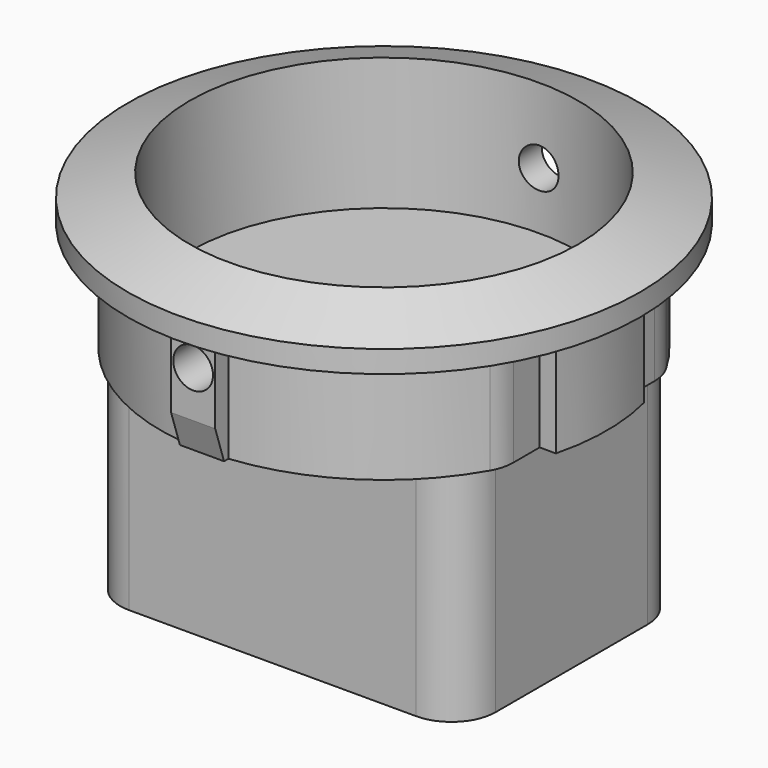
from build123d import *

# Parameters (mm, degrees)
F0_R      = 11.6
F1_DEPTH  = 2
F3_DEPTH  = 5
F5_DEPTH  = 10
F6_W      = 0.8
F6_H      = 5
F7_DEPTH  = 5
F8_R      = 8.8
F9_DEPTH  = 6
F10_SIZE2 = 0.99999
F10_SIZE  = 2.79999
F11_R     = 2
F12_SIZE2 = 0.5
F12_SIZE  = 1.5
F13_R     = 0.9
F14_DEPTH = 22.4013731274


# Not quite as in the source:
# - a fillet or chamfer is up to 0.001 mm smaller than in the source, because OpenCascade refuses the exact size


with BuildPart() as f1:
    # F0 (on Top) → F1 (new body)
    with BuildSketch(Plane.XY):
        Circle(F0_R)
    extrude(amount=F1_DEPTH)

    # F2 (on face) → F3 (join)
    with BuildSketch(Plane(origin=(0, 0, 0), x_dir=(1, 0, 0), z_dir=(0, 0, -1))):
        with BuildLine():
            Line((-9.05, -2.5), (-9.05, -4.4841387133))
            ThreePointArc((-9.05, -4.4841387133), (0, -10.1), (9.05, -4.4841387133))
            Line((9.05, -4.4841387133), (9.05, -2.5))
            Line((9.05, -2.5), (9.05, 2.5))
            Line((9.05, 2.5), (9.05, 4.4841387133))
            ThreePointArc((9.05, 4.4841387133), (5.7442463725, 8.3074444694), (1, 10.0503731274))
            Line((1, 10.0503731274), (1, 10.8003731274))
            Line((1, 10.8003731274), (-1, 10.8003731274))
            Line((-1, 10.8003731274), (-1, 10.0503731274))
            ThreePointArc((-1, 10.0503731274), (-5.7442463725, 8.3074444694), (-9.05, 4.4841387133))
            Line((-9.05, 4.4841387133), (-9.05, 2.5))
            Line((-9.05, 2.5), (-9.05, -2.5))
        make_face()
        with BuildLine():
            Line((-9.7857038582, -2.5), (-9.05, -2.5))
            Line((-9.05, -2.5), (-9.05, 2.5))
            Line((-9.05, 2.5), (-9.7857038582, 2.5))
            ThreePointArc((-9.7857038582, 2.5), (-10.1, 0), (-9.7857038582, -2.5))
        make_face()
        with BuildLine():
            Line((9.05, 2.5), (9.05, -2.5))
            Line((9.05, -2.5), (9.7857038582, -2.5))
            ThreePointArc((9.7857038582, -2.5), (10.1, 0), (9.7857038582, 2.5))
            Line((9.7857038582, 2.5), (9.05, 2.5))
        make_face()
    extrude(amount=F3_DEPTH)

    # F4 (on face) → F5 (join)
    with BuildSketch(Plane(origin=(0, 0, -5), x_dir=(1, 0, 0), z_dir=(0, 0, -1))):
        with BuildLine():
            Line((6.5, 6.3), (-6.5, 6.3))
            ThreePointArc((-6.5, 6.3), (-7.9142135624, 5.7142135624), (-8.5, 4.3))
            Line((-8.5, 4.3), (-8.5, -4.3))
            ThreePointArc((-8.5, -4.3), (-7.9142135624, -5.7142135624), (-6.5, -6.3))
            Line((-6.5, -6.3), (6.5, -6.3))
            ThreePointArc((6.5, -6.3), (7.9142135624, -5.7142135624), (8.5, -4.3))
            Line((8.5, -4.3), (8.5, 4.3))
            ThreePointArc((8.5, 4.3), (7.9142135624, 5.7142135624), (6.5, 6.3))
        make_face()
    extrude(amount=F5_DEPTH)

    # F6 (on face) → F7 (cut)
    with BuildSketch(Plane(origin=(0, 0, -15), x_dir=(1, 0, 0), z_dir=(0, 0, -1))):
        Rectangle(F6_W, F6_H)
        with Locations((-7.35, 0)):
            Rectangle(F6_W, F6_H)
        with Locations((7.35, 0)):
            Rectangle(F6_W, F6_H)
    extrude(amount=-F7_DEPTH, mode=Mode.SUBTRACT)

    # F8 (on face) → F9 (cut)
    with BuildSketch(Plane.XY.offset(2)):
        Circle(F8_R)
    extrude(amount=-F9_DEPTH, mode=Mode.SUBTRACT)

    # F10 (size 2.8 and 1 in the source; OpenCascade refuses exactly that, so slightly less here)
    f10_edges = [f1.edges().sort_by_distance(p)[0] for p in [
        (-11.6, 0, 2),
    ]]
    f10_side = f1.faces().sort_by_distance((-11.271902, 0, 2))[0]
    chamfer(f10_edges, length=F10_SIZE, length2=F10_SIZE2, reference=f10_side)

    # F11
    f11_edges = [f1.edges().sort_by_distance(p)[0] for p in [
        (-9.05, 4.484139, -2.5),
        (-9.05, -4.484139, -2.5),
        (9.05, -4.484139, -2.5),
        (9.05, 4.484139, -2.5),
    ]]
    fillet(f11_edges, radius=F11_R)

    # F12
    f12_edges = [f1.edges().sort_by_distance(p)[0] for p in [
        (0, -10.800373, -5),
    ]]
    f12_side = f1.faces().sort_by_distance((0, -10.800373, -2.5))[0]
    chamfer(f12_edges, length=F12_SIZE, length2=F12_SIZE2, reference=f12_side)

    # F13 (on face) → F14 (cut, through all)
    with BuildSketch(Plane.XZ.offset(10.8003731274)):
        with Locations((0, -1.4)):
            Circle(F13_R)
    extrude(amount=-F14_DEPTH, mode=Mode.SUBTRACT)


solid = f1.part
